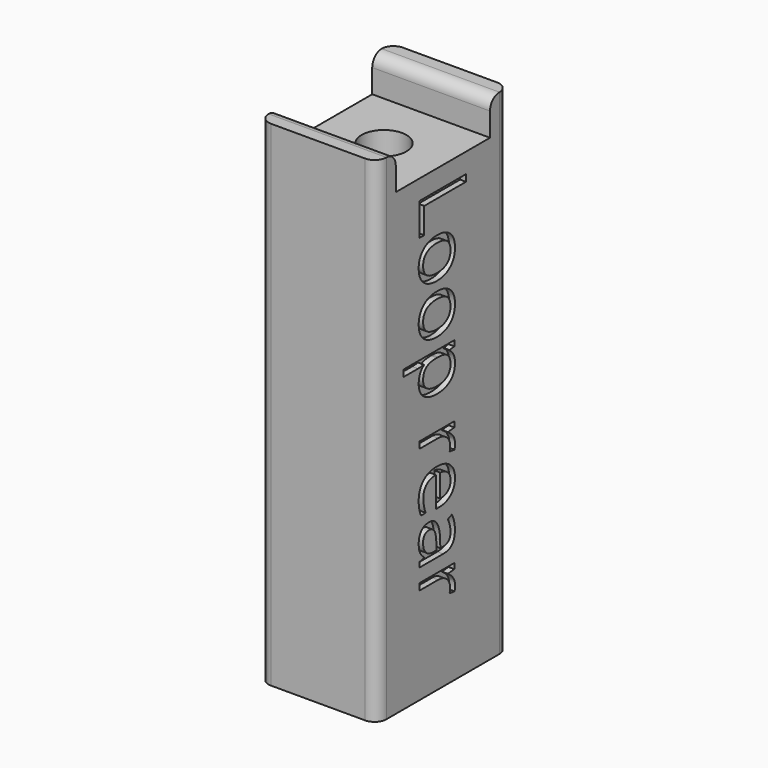
from build123d import *

# Parameters (mm, degrees)
F0_W         = 10
F0_H         = 14
F0_R         = 1.9
F1_DEPTH     = 39
F2_W         = 10
F2_H         = 2
F3_DEPTH     = 3
F4_R         = 0.99999
F5_TEXT_SIZE = 6.9444444444
F6_DEPTH     = 0.5


# Not quite as in the source:
# - a fillet or chamfer is up to 0.001 mm smaller than in the source, because OpenCascade refuses the exact size
# - Text() gives the source's letters only with a copy of the font that has no kerning and outlines rounded to 1/6400 em; it was checked with that copy


with BuildPart() as f1:
    # F0 (on Top) → F1 (new body)
    with BuildSketch(Plane.XY):
        Rectangle(F0_W, F0_H)
        Circle(F0_R, mode=Mode.SUBTRACT)
    extrude(amount=F1_DEPTH)

    # F2 (on face) → F3 (join)
    with BuildSketch(Plane.XY.offset(39)):
        with Locations((0, 6)):
            Rectangle(F2_W, F2_H)
        with Locations((0, -6)):
            Rectangle(F2_W, F2_H)
    extrude(amount=F3_DEPTH)

    # F4 (radius 1 in the source; OpenCascade refuses exactly that, so slightly less here)
    f4_edges = [f1.edges().sort_by_distance(p)[0] for p in [
        (5, -7, 21),
        (-5, -7, 21),
        (5, 7, 21),
        (-5, 7, 21),
        (0, 5, 42),
        (0, -5, 42),
    ]]
    fillet(f4_edges, radius=F4_R)

    # F5 (on face) → F6 (cut)
    with BuildSketch(Plane.YZ.offset(5)):
        with Locations(Location((-2.5, 38), (0, 0, -90))):
            Text('Loop rear', F5_TEXT_SIZE, font='Open Sans', text_align=(TextAlign.LEFT, TextAlign.BOTTOM))
    extrude(amount=-F6_DEPTH, mode=Mode.SUBTRACT)


solid = f1.part
